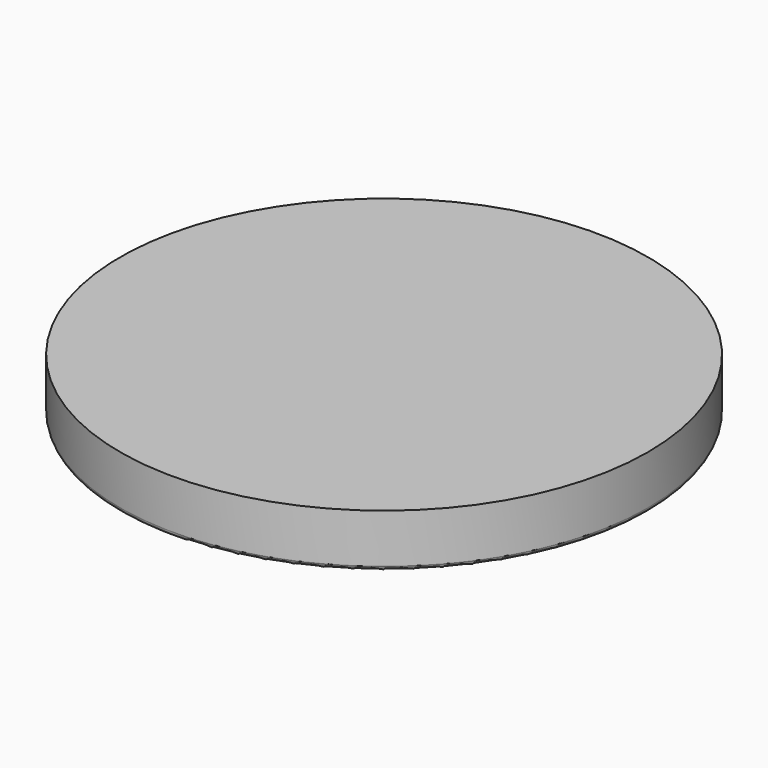
from build123d import *

# Parameters (mm, degrees)
F0_R         = 11.6
F1_DEPTH     = 2.15
F2_R         = 11.6
F2_TEXT_SIZE = 5.9955033725
F1_FACE1_R   = 11.6
F3_DEPTH     = 0.2
F4_R         = 0.2


# Not quite as in the source:
# - Text() gives the source's letters only with a copy of the font that has no kerning and outlines rounded to 1/6400 em; it was checked with that copy


with BuildPart() as f1:
    # F0 (on Top) → F1 (new body)
    with BuildSketch(Plane.XY):
        Circle(F0_R)
    extrude(amount=F1_DEPTH)

    # F2 (on face) + F1_face1 (on face) → F3 (join)
    with BuildSketch(Plane.XY.offset(2.15)):
        Circle(F2_R)
        with BuildLine():
            Line((-4.3466062745, 2.4520212206), (-5.2515525647, -1.8282061089))
            Line((-5.2515525647, -1.8282061089), (-6.1443204888, -1.8282061089))
            Line((-6.1443204888, -1.8282061089), (-5.6178403489, 0.5990359595))
            add(Edge.make_bspline(
                [(-5.6178403489, 0.5990359595), (-5.5147926347, 1.0440147255), (-5.3948825672, 1.4393432291)],
                knots=[0, 0, 0, 1, 1, 1], degree=2))
            add(Edge.make_bspline(
                [(-5.3948825672, 1.4393432291), (-5.4211128945, 1.415923294), (-5.5747476684, 1.301634011)],
                knots=[0, 0, 0, 1, 1, 1], degree=2))
            add(Edge.make_bspline(
                [(-5.5747476684, 1.301634011), (-5.7283824423, 1.187344728), (-6.3438583354, 0.8032577932)],
                knots=[0, 0, 0, 1, 1, 1], degree=2))
            Line((-6.3438583354, 0.8032577932), (-6.7326292572, 1.4327856473))
            Line((-6.7326292572, 1.4327856473), (-5.0754346532, 2.4520212206))
            Line((-5.0754346532, 2.4520212206), (-4.3466062745, 2.4520212206))
        make_face(mode=Mode.SUBTRACT)
        with BuildLine():
            add(Edge.make_bspline(
                [(-0.9127753976, 1.7082040835), (-1.1146552377, 1.7634751302), (-1.3141930844, 1.7634751302)],
                knots=[0, 0, 0, 1, 1, 1], degree=2))
            add(Edge.make_bspline(
                [(-1.3141930844, 1.7634751302), (-1.700153614, 1.7634751302), (-2.0092967566, 1.5264653875)],
                knots=[0, 0, 0, 1, 1, 1], degree=2))
            add(Edge.make_bspline(
                [(-2.0092967566, 1.5264653875), (-2.3184398992, 1.2894556448), (-2.5057993796, 0.828551323)],
                knots=[0, 0, 0, 1, 1, 1], degree=2))
            add(Edge.make_bspline(
                [(-2.5057993796, 0.828551323), (-2.69315886, 0.3676470013), (-2.69315886, -0.1625803282)],
                knots=[0, 0, 0, 1, 1, 1], degree=2))
            add(Edge.make_bspline(
                [(-2.69315886, -0.1625803282), (-2.69315886, -0.6515885721), (-2.492684216, -0.8885983147)],
                knots=[0, 0, 0, 1, 1, 1], degree=2))
            add(Edge.make_bspline(
                [(-2.492684216, -0.8885983147), (-2.292209572, -1.1256080574), (-1.8528515905, -1.1256080574)],
                knots=[0, 0, 0, 1, 1, 1], degree=2))
            add(Edge.make_bspline(
                [(-1.8528515905, -1.1256080574), (-1.4256719752, -1.1256080574), (-0.863593534, -0.8998398836)],
                knots=[0, 0, 0, 1, 1, 1], degree=2))
            Line((-0.863593534, -0.8998398836), (-0.863593534, -1.6614561714))
            add(Edge.make_bspline(
                [(-0.863593534, -1.6614561714), (-1.4453447206, -1.8872243452), (-2.0345902865, -1.8872243452)],
                knots=[0, 0, 0, 1, 1, 1], degree=2))
            add(Edge.make_bspline(
                [(-2.0345902865, -1.8872243452), (-2.7774706262, -1.8872243452), (-3.1905982805, -1.4492715598)],
                knots=[0, 0, 0, 1, 1, 1], degree=2))
            add(Edge.make_bspline(
                [(-3.1905982805, -1.4492715598), (-3.6037259347, -1.0113187744), (-3.6037259347, -0.2094201983)],
                knots=[0, 0, 0, 1, 1, 1], degree=2))
            add(Edge.make_bspline(
                [(-3.6037259347, -0.2094201983), (-3.6037259347, 0.5578168739), (-3.2992667791, 1.2032702838)],
                knots=[0, 0, 0, 1, 1, 1], degree=2))
            add(Edge.make_bspline(
                [(-3.2992667791, 1.2032702838), (-2.9948076235, 1.8487236937), (-2.4851898368, 2.1840971636)],
                knots=[0, 0, 0, 1, 1, 1], degree=2))
            add(Edge.make_bspline(
                [(-2.4851898368, 2.1840971636), (-1.9755720501, 2.5194706335), (-1.3141930844, 2.5194706335)],
                knots=[0, 0, 0, 1, 1, 1], degree=2))
            add(Edge.make_bspline(
                [(-1.3141930844, 2.5194706335), (-0.9479053002, 2.5194706335), (-0.6640556874, 2.4534264167)],
                knots=[0, 0, 0, 1, 1, 1], degree=2))
            add(Edge.make_bspline(
                [(-0.6640556874, 2.4534264167), (-0.3802060746, 2.3873821999), (-0.0551373761, 2.2122010857)],
                knots=[0, 0, 0, 1, 1, 1], degree=2))
            Line((-0.0551373761, 2.2122010857), (-0.4008156175, 1.4796255174))
            add(Edge.make_bspline(
                [(-0.4008156175, 1.4796255174), (-0.7108955575, 1.6529330367), (-0.9127753976, 1.7082040835)],
                knots=[0, 0, 0, 1, 1, 1], degree=2))
        make_face(mode=Mode.SUBTRACT)
        Polygon((3.932809164, 2.4520212206), (3.0278628737, -1.8282061089), (2.1322845574, -1.8282061089), (2.5238658714, 0.0191583677), (1.1458368932, 0.0191583677), (0.7533187817, -1.8282061089), (-0.1394491423, -1.8282061089), (0.7645603506, 2.4520212206), (1.6610754642, 2.4520212206), (1.3060292489, 0.7742170737), (2.6849950246, 0.7742170737), (3.0391044425, 2.4520212206), align=None, mode=Mode.SUBTRACT)
        Polygon((5.3052173578, -0.136350001), (4.9511079399, -1.8282061089), (4.0583400158, -1.8282061089), (4.9623495087, 2.4520212206), (7.3455620993, 2.4520212206), (7.1872433383, 1.7082040835), (5.7005458614, 1.7082040835), (5.4691569032, 0.604656744), (6.8537434632, 0.604656744), (6.6898039179, -0.136350001), align=None, mode=Mode.SUBTRACT)
        with Locations((-7.2656669789, -1.8282061089)):
            Text('1CHF', F2_TEXT_SIZE, font='Open Sans', font_style=FontStyle.BOLDITALIC, text_align=(TextAlign.LEFT, TextAlign.BOTTOM))
    with BuildSketch(Plane(origin=(0, 0, 0), x_dir=(1, 0, 0), z_dir=(0, 0, -1))):
        Circle(F1_FACE1_R)
    extrude(amount=F3_DEPTH, dir=(0, 0, 1))

    # F4
    f4_edges = [f1.edges().sort_by_distance(p)[0] for p in [
        (-11.6, 0, 0),
    ]]
    fillet(f4_edges, radius=F4_R)


solid = f1.part
